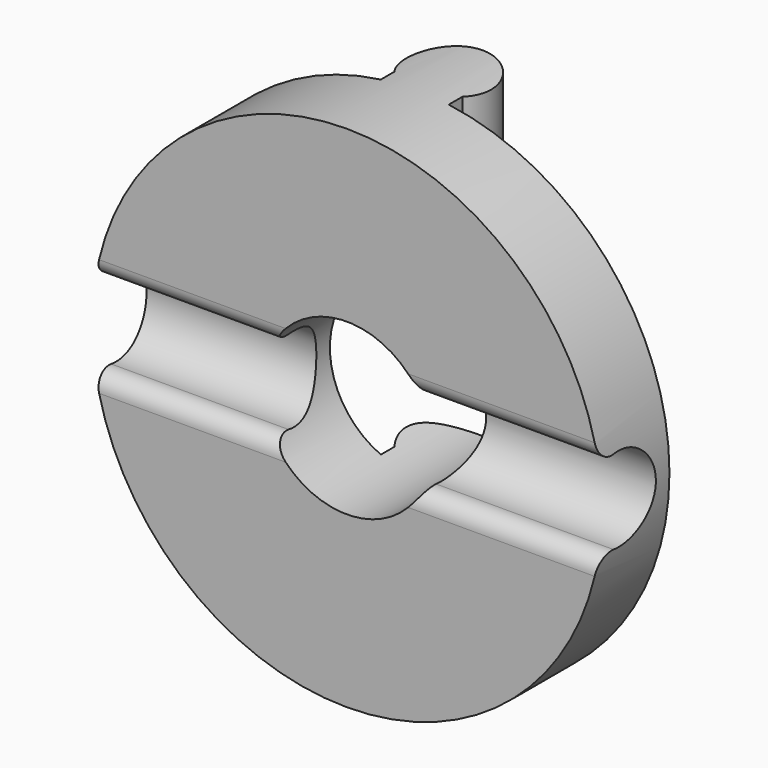
from build123d import *

# Parameters (mm, degrees)
F0_R          = 1.5
F1_DEPTH      = 1
F3_DEPTH      = 1.501
F3_DEPTH_BACK = 25
F4_R          = 0.25
F5_DEPTH      = 1.5010001
F5_DEPTH_BACK = 25
F6_T1_DEPTH   = 3.705264557
F7_R          = 0.5
F8_DEPTH      = 1.0010001
F10_DEPTH     = 0.1


# Not quite as in the source:
# - a fillet or chamfer that OpenCascade refuses, or shapes differently, is made with other operations: its cross-section is extruded or revolved along the edge and cut away or added


with BuildPart() as f1:
    # F0 (on Front) → F1 (new body)
    with BuildSketch(Plane.XZ):
        Circle(F0_R)
    extrude(amount=F1_DEPTH)

    # F2 (on Top) → F3 (cut, two sides)
    with BuildSketch(Plane.XY) as f3_sk:
        with BuildLine():
            ThreePointArc((-0.2, -0.4), (0, 0), (0.2, -0.4))
            Line((0.2, -0.4), (1.99, -0.4))
            Line((1.99, -0.4), (1.99, 0.99))
            Line((1.99, 0.99), (-1.99, 0.99))
            Line((-1.99, 0.99), (-1.99, -0.4))
            Line((-1.99, -0.4), (-0.2, -0.4))
        make_face()
    extrude(amount=-F3_DEPTH, mode=Mode.SUBTRACT)
    extrude(f3_sk.sketch, amount=F3_DEPTH_BACK, mode=Mode.SUBTRACT)

    # F4 (on Right) → F5 (cut, two sides)
    with BuildSketch(Plane.YZ) as f5_sk:
        with Locations((-0.85, 0)):
            Circle(F4_R)
    extrude(amount=-F5_DEPTH, mode=Mode.SUBTRACT)
    extrude(f5_sk.sketch, amount=F5_DEPTH_BACK, mode=Mode.SUBTRACT)

    # F6: fillet of radius 0.1 on 2 edges, made by hand

    # F6_s2 → F6_t1 (cut)
    with BuildSketch(Plane.YZ.offset(-1.8526322785)):
        with BuildLine():
            ThreePointArc((-1, -0.3464101615), (-0.9654653671, -0.2708172669), (-0.8857142857, -0.2474358297))
            ThreePointArc((-0.8857142857, -0.2474358297), (-0.9458383455, -0.2309004364), (-1, -0.2))
            Line((-1, -0.2), (-1, -0.3464101615))
        make_face()
        with BuildLine():
            ThreePointArc((-1, 0.3464101615), (-0.9654653671, 0.2708172669), (-0.8857142857, 0.2474358297))
            ThreePointArc((-0.8857142857, 0.2474358297), (-0.9458383455, 0.2309004364), (-1, 0.2))
            Line((-1, 0.2), (-1, 0.3464101615))
        make_face()
    extrude(amount=F6_T1_DEPTH, mode=Mode.SUBTRACT)

    # F7 (on Front) → F8 (cut, through all)
    with BuildSketch(Plane.XZ):
        Circle(F7_R)
    extrude(amount=F8_DEPTH, mode=Mode.SUBTRACT)

    # F9 (on face) → F10 (cut)
    with BuildSketch(Plane(origin=(0, -0.4, 0), x_dir=(-1, 0, 0), z_dir=(0, 1, 0))):
        with BuildLine():
            ThreePointArc((0.2, 0.4582575695), (0.5, 0), (0.2, -0.4582575695))
            Line((0.2, -0.4582575695), (0.2, -1.4866068747))
            ThreePointArc((0.2, -1.4866068747), (1.5, 0), (0.2, 1.4866068747))
            Line((0.2, 1.4866068747), (0.2, 0.4582575695))
        make_face()
        with BuildLine():
            ThreePointArc((-0.2, -0.4582575695), (-0.5, 0), (-0.2, 0.4582575695))
            Line((-0.2, 0.4582575695), (-0.2, 1.4866068747))
            ThreePointArc((-0.2, 1.4866068747), (-1.5, 0), (-0.2, -1.4866068747))
            Line((-0.2, -1.4866068747), (-0.2, -0.4582575695))
        make_face()
    extrude(amount=-F10_DEPTH, mode=Mode.SUBTRACT)


solid = f1.part
